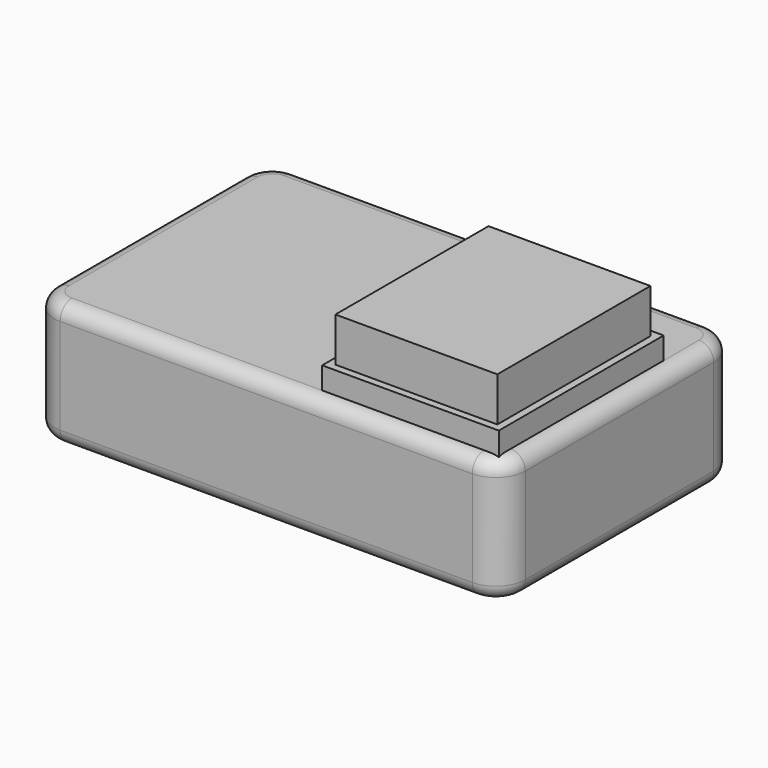
from build123d import *

# Parameters (mm, degrees)
F0_W         = 32
F0_H         = 20
F0_W_2       = 12
F0_H_2       = 14
F0_R         = 1.25
F0_W_3       = 11
F0_H_3       = 13
F1_DEPTH     = 8.5
F2_DEPTH     = 5
F3_R         = 2
F4_DEPTH     = 13
F5_DEPTH     = 10
F6_T1_DEPTH  = 28
F6_T3_DEPTH  = 16
F6_T6_ANGLE  = 90
F6_T8_ANGLE  = 90
F6_T10_ANGLE = 90
F6_T12_ANGLE = 90
F6_T14_ANGLE = 90
F6_T16_ANGLE = 90
F6_T20_ANGLE = 90
F6_T26_ANGLE = 90
F6_T32_ANGLE = 90
F6_T36_ANGLE = 90


# Not quite as in the source:
# - a fillet or chamfer that OpenCascade refuses, or shapes differently, is made with other operations: its cross-section is extruded or revolved along the edge and cut away or added


with BuildPart() as f1:
    # F0 (on Top) → F1 (new body)
    with BuildSketch(Plane.XY):
        Rectangle(F0_W, F0_H)
        with Locations((9, -2)):
            Rectangle(F0_W_2, F0_H_2, mode=Mode.SUBTRACT)
        with Locations((9.5, 7)):
            Circle(F0_R, mode=Mode.SUBTRACT)
        with Locations((9, -2)):
            Rectangle(F0_W_2, F0_H_2)
        with Locations((9, -2)):
            Rectangle(F0_W_3, F0_H_3, mode=Mode.SUBTRACT)
        with Locations((9, -2)):
            Rectangle(F0_W_3, F0_H_3)
    extrude(amount=F1_DEPTH)

    # F0 (on Top) → F2 (join)
    with BuildSketch(Plane.XY):
        with Locations((9.5, 7)):
            Circle(F0_R)
    extrude(amount=F2_DEPTH)

    # F3
    f3_edges = [f1.edges().sort_by_distance(p)[0] for p in [
        (-16, 10, 4.25),
        (-16, -10, 4.25),
        (16, -10, 4.25),
        (16, 10, 4.25),
    ]]
    fillet(f3_edges, radius=F3_R)

    # F0 (on Top) → F4 (join)
    with BuildSketch(Plane.XY):
        with Locations((9, -2)):
            Rectangle(F0_W_3, F0_H_3)
    extrude(amount=F4_DEPTH)

    # F0 (on Top) → F5 (join)
    with BuildSketch(Plane.XY):
        with Locations((9, -2)):
            Rectangle(F0_W_2, F0_H_2)
        with Locations((9, -2)):
            Rectangle(F0_W_3, F0_H_3, mode=Mode.SUBTRACT)
    extrude(amount=F5_DEPTH)

    # F6: fillet of radius 1 on 18 edges, made by hand

    # F6_s2 → F6_t1 (cut)
    with BuildSketch(Plane.YZ.offset(-14)):
        with BuildLine():
            ThreePointArc((-9, 0), (-9.7071067812, 0.2928932188), (-10, 1))
            Line((-10, 1), (-10, 0))
            Line((-10, 0), (-9, 0))
        make_face()
        with BuildLine():
            ThreePointArc((-9, 8.5), (-9.7071067812, 8.2071067812), (-10, 7.5))
            Line((-10, 7.5), (-10, 8.5))
            Line((-10, 8.5), (-9, 8.5))
        make_face()
        with BuildLine():
            ThreePointArc((10, 1), (9.7071067812, 0.2928932188), (9, 0))
            Line((9, 0), (10, 0))
            Line((10, 0), (10, 1))
        make_face()
        with BuildLine():
            ThreePointArc((10, 7.5), (9.7071067812, 8.2071067812), (9, 8.5))
            Line((9, 8.5), (10, 8.5))
            Line((10, 8.5), (10, 7.5))
        make_face()
    extrude(amount=F6_T1_DEPTH, mode=Mode.SUBTRACT)

    # F6_s4 → F6_t3 (cut)
    with BuildSketch(Plane.XZ.offset(-8)):
        with BuildLine():
            ThreePointArc((-15, 0), (-15.7071067812, 0.2928932188), (-16, 1))
            Line((-16, 1), (-16, 0))
            Line((-16, 0), (-15, 0))
        make_face()
        with BuildLine():
            ThreePointArc((15, 0), (15.7071067812, 0.2928932188), (16, 1))
            Line((16, 1), (16, 0))
            Line((16, 0), (15, 0))
        make_face()
        with BuildLine():
            ThreePointArc((15, 8.5), (15.7071067812, 8.2071067812), (16, 7.5))
            Line((16, 7.5), (16, 8.5))
            Line((16, 8.5), (15, 8.5))
        make_face()
        with BuildLine():
            ThreePointArc((-15, 8.5), (-15.7071067812, 8.2071067812), (-16, 7.5))
            Line((-16, 7.5), (-16, 8.5))
            Line((-16, 8.5), (-15, 8.5))
        make_face()
    extrude(amount=F6_T3_DEPTH, mode=Mode.SUBTRACT)

    # F6_s5 → F6_t6 (revolve, cut)
    with BuildSketch(Plane.YZ.offset(-14)):
        with BuildLine():
            ThreePointArc((9, 0), (9.7071067812, 0.2928932188), (10, 1))
            Line((10, 1), (10, 0))
            Line((10, 0), (9, 0))
        make_face()
    revolve(axis=Axis((-14, 8, 0), (0, 0, 1)), revolution_arc=F6_T6_ANGLE, mode=Mode.SUBTRACT)

    # F6_s7 → F6_t8 (revolve, cut)
    with BuildSketch(Plane.XZ.offset(8)):
        with BuildLine():
            ThreePointArc((-15, 0), (-15.7071067812, 0.2928932188), (-16, 1))
            Line((-16, 1), (-16, 0))
            Line((-16, 0), (-15, 0))
        make_face()
    revolve(axis=Axis((-14, -8, 0), (0, 0, 1)), revolution_arc=F6_T8_ANGLE, mode=Mode.SUBTRACT)

    # F6_s9 → F6_t10 (revolve, cut)
    with BuildSketch(Plane.XZ.offset(8)):
        with BuildLine():
            ThreePointArc((15, 0), (15.7071067812, 0.2928932188), (16, 1))
            Line((16, 1), (16, 0))
            Line((16, 0), (15, 0))
        make_face()
    revolve(axis=Axis((14, -8, 0), (0, 0, -1)), revolution_arc=F6_T10_ANGLE, mode=Mode.SUBTRACT)

    # F6_s11 → F6_t12 (revolve, cut)
    with BuildSketch(Plane.YZ.offset(14)):
        with BuildLine():
            ThreePointArc((9, 0), (9.7071067812, 0.2928932188), (10, 1))
            Line((10, 1), (10, 0))
            Line((10, 0), (9, 0))
        make_face()
    revolve(axis=Axis((14, 8, 0), (0, 0, -1)), revolution_arc=F6_T12_ANGLE, mode=Mode.SUBTRACT)

    # F6_s13 → F6_t14 (revolve, cut)
    with BuildSketch(Plane.YZ.offset(14)):
        with BuildLine():
            ThreePointArc((10, 7.5), (9.7071067812, 8.2071067812), (9, 8.5))
            Line((9, 8.5), (10, 8.5))
            Line((10, 8.5), (10, 7.5))
        make_face()
    revolve(axis=Axis((14, 8, 8.5), (0, 0, -1)), revolution_arc=F6_T14_ANGLE, mode=Mode.SUBTRACT)

    # F6_s15 → F6_t16 (revolve, cut)
    with BuildSketch(Plane.YZ.offset(-14)):
        with BuildLine():
            ThreePointArc((10, 7.5), (9.7071067812, 8.2071067812), (9, 8.5))
            Line((9, 8.5), (10, 8.5))
            Line((10, 8.5), (10, 7.5))
        make_face()
    revolve(axis=Axis((-14, 8, 8.5), (0, 0, 1)), revolution_arc=F6_T16_ANGLE, mode=Mode.SUBTRACT)


with BuildPart() as f6_tool18:
    # F6_s19 → F6_t20 (revolve)
    with BuildSketch(Plane.XZ.offset(8)):
        with BuildLine():
            ThreePointArc((15, 8.5), (15.7071067812, 8.2071067812), (16, 7.5))
            Line((16, 7.5), (16, 8.5))
            Line((16, 8.5), (15, 8.5))
        make_face()
    revolve(axis=Axis((14, -8, 8.5), (0, 0, -1)), revolution_arc=F6_T20_ANGLE)

    split(bisect_by=Plane.YZ.offset(15), keep=Keep.TOP)

    split(bisect_by=Plane.XZ.offset(9), keep=Keep.BOTTOM)


with BuildPart() as f1_1:
    add(f1.part)

    # F6_t17: cut F6_tool18
    add(f6_tool18.part, mode=Mode.SUBTRACT)


with BuildPart() as f6_tool24:
    # F6_s25 → F6_t26 (revolve)
    with BuildSketch(Plane.XZ.offset(8)):
        with BuildLine():
            ThreePointArc((15, 8.5), (15.7071067812, 8.2071067812), (16, 7.5))
            Line((16, 7.5), (16, 8.5))
            Line((16, 8.5), (15, 8.5))
        make_face()
    revolve(axis=Axis((14, -8, 8.5), (0, 0, -1)), revolution_arc=F6_T26_ANGLE)

    split(bisect_by=Plane.YZ.offset(15), keep=Keep.BOTTOM)

    split(bisect_by=Plane.XZ.offset(9), keep=Keep.TOP)


with BuildPart() as f1_2:
    add(f1_1.part)

    # F6_t23: cut F6_tool24
    add(f6_tool24.part, mode=Mode.SUBTRACT)


with BuildPart() as f6_tool30:
    # F6_s31 → F6_t32 (revolve)
    with BuildSketch(Plane.XZ.offset(8)):
        with BuildLine():
            ThreePointArc((15, 8.5), (15.7071067812, 8.2071067812), (16, 7.5))
            Line((16, 7.5), (16, 8.5))
            Line((16, 8.5), (15, 8.5))
        make_face()
    revolve(axis=Axis((14, -8, 8.5), (0, 0, -1)), revolution_arc=F6_T32_ANGLE)

    split(bisect_by=Plane.YZ.offset(15), keep=Keep.TOP)

    split(bisect_by=Plane.XZ.offset(9), keep=Keep.TOP)


with BuildPart() as f1_3:
    add(f1_2.part)

    # F6_t29: cut F6_tool30
    add(f6_tool30.part, mode=Mode.SUBTRACT)

    # F6_s35 → F6_t36 (revolve, cut)
    with BuildSketch(Plane.XZ.offset(8)):
        with BuildLine():
            ThreePointArc((-15, 8.5), (-15.7071067812, 8.2071067812), (-16, 7.5))
            Line((-16, 7.5), (-16, 8.5))
            Line((-16, 8.5), (-15, 8.5))
        make_face()
    revolve(axis=Axis((-14, -8, 8.5), (0, 0, 1)), revolution_arc=F6_T36_ANGLE, mode=Mode.SUBTRACT)


solid = f1_3.part
